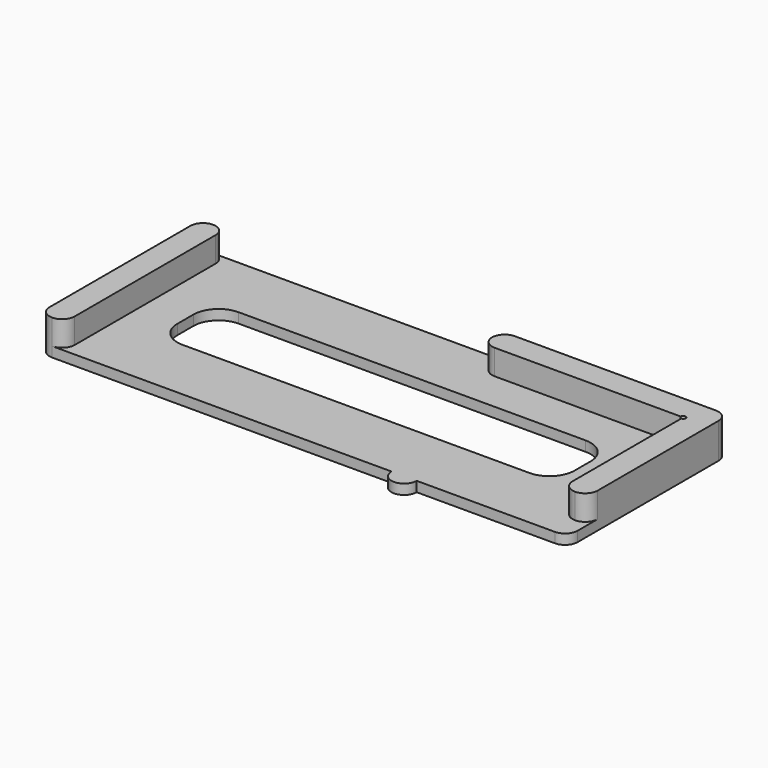
from build123d import *

# Parameters (mm, degrees)
F4_W     = 3
F4_H     = 1
F6_R     = 1
F7_R     = 0.49999
F8_R     = 0.1
F9_DEPTH = 1


# Not quite as in the source:
# - a fillet or chamfer is up to 0.001 mm smaller than in the source, because OpenCascade refuses the exact size


with BuildPart() as f3:
    # F3: sweep along a path in F1
    with BuildLine(Plane.XZ) as f3_path:
        Line((0, 0), (0, -0.4))
    # F2 (on Top) → F3 (sweep)
    with BuildSketch(Plane.XY):
        Polygon((10.5, -7), (10.5, 1), (4.5, 1), (3.5, 1), (-10.5, 1), (-10.5, -7), (3.5, -7), (4.5, -7), align=None)
        Polygon((-7.9, -4.4), (-7.9, -1.6), (-4.5, -1.6), (4.5, -1.6), (7.9, -1.6), (7.9, -4.4), align=None, mode=Mode.SUBTRACT)
        with BuildLine():
            Line((3.5, 1), (4.5, 1))
            ThreePointArc((4.5, 1), (4, 1.5), (3.5, 1))
        make_face()
        with BuildLine():
            ThreePointArc((3.5, -7), (4, -7.5), (4.5, -7))
            Line((4.5, -7), (3.5, -7))
        make_face()
    sweep(path=f3_path.line)

    # F5: sweep along a path in F1
    with BuildLine(Plane.XZ) as f5_path:
        Line((0, 0), (0, 1))
    # F4 (on face) → F5 (sweep)
    with BuildSketch(Plane.XY):
        Polygon((4.5, 0), (9.5, 0), (9.5, -6), (10.5, -6), (10.5, 1), (4.5, 1), align=None)
        with Locations((3, 0.5)):
            Rectangle(F4_W, F4_H)
        Polygon((-9.5, -6), (-9.5, 0), (-9.5, 1), (-10.5, 1), (-10.5, -7), (-9.5, -7), align=None)
    sweep(path=f5_path.line)

    # F6
    f6_edges = [f3.edges().sort_by_distance(p)[0] for p in [
        (-7.9, -1.6, -0.2),
        (-7.9, -4.4, -0.2),
        (7.9, -1.6, -0.2),
        (7.9, -4.4, -0.2),
    ]]
    fillet(f6_edges, radius=F6_R)

    # F7 (radius 0.5 in the source; OpenCascade refuses exactly that, so slightly less here)
    f7_edges = [f3.edges().sort_by_distance(p)[0] for p in [
        (-10.5, -7, 0.3),
        (-10.5, 1, 0.3),
        (9.5, -6, 0.5),
        (10.5, -6, 0.5),
        (1.5, 0, 0.5),
        (10.5, -7, -0.2),
        (10.5, 1, 0.3),
        (1.5, 1, 0.5),
        (-9.5, 1, 0.5),
        (-9.5, -7, 0.5),
    ]]
    fillet(f7_edges, radius=F7_R)

    # F8 (on face) → F9 (cut, through all)
    with BuildSketch(Plane.XY.offset(1)):
        with Locations((9.5, 0)):
            Circle(F8_R)
    extrude(amount=-F9_DEPTH, mode=Mode.SUBTRACT)


solid = f3.part
